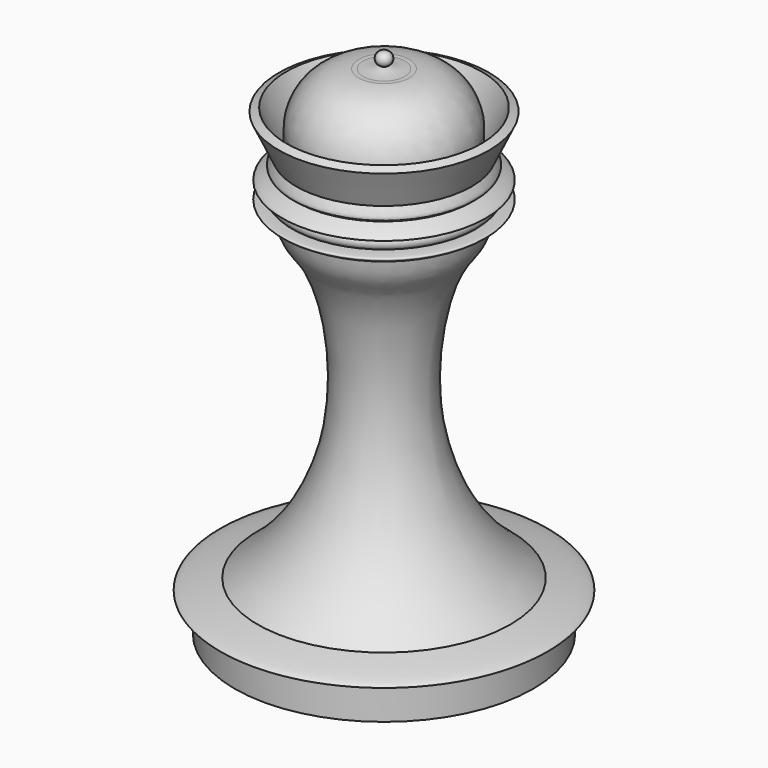
from build123d import *

# Parameters (mm, degrees)
F0_W = 22.86
F0_H = 5.08


# Not quite as in the source:
# - a fillet or chamfer that OpenCascade refuses, or shapes differently, is made with other operations: its cross-section is extruded or revolved along the edge and cut away or added
# - ends of sketch curves that miss each other by under 0.0002 mm in the source are joined


with BuildPart() as f1:
    # F0 (on Front) → F1 (revolve)
    with BuildSketch(Plane.XZ):
        with BuildLine():
            Line((0, 55.7105094194), (0, 0))
            Line((0, 0), (22.86, 0))
            add(Edge.make_bspline(
                [(22.86, 0), (21.5989604618, 0.7698820082), (20.4285707435, 1.5817251932), (19.3433039435, 2.4293450133)],
                knots=[0, 0, 0, 0, 0.0399308158, 0.0399308158, 0.0399308158, 0.0399308158], degree=3))
            add(Edge.make_bspline(
                [(19.3433039435, 2.4293450133), (2.1960366332, 15.8217786838), (8.0106373207, 47.4585030975), (12.7210086452, 48.040195095), (13.216347906, 51.9578989549)],
                knots=[0.0399308158, 0.0399308158, 0.0399308158, 0.0399308158, 0.6708396138, 0.9340401236, 0.9340401236, 0.9340401236, 0.9340401236], degree=3))
            add(Edge.make_bspline(
                [(13.216347906, 51.9578989549), (13.2835273481, 52.4892300656), (13.3343132727, 53.0894723366), (13.3667210402, 53.7746848436)],
                knots=[0.9340401236, 0.9340401236, 0.9340401236, 0.9340401236, 0.9697361905, 0.9697361905, 0.9697361905, 0.9697361905], degree=3))
            add(Edge.make_bspline(
                [(13.3667210402, 53.7746848436), (13.3941969664, 54.3556211357), (13.4084627224, 54.9976338064), (13.4083088487, 55.7105094194)],
                knots=[0.9697361905, 0.9697361905, 0.9697361905, 0.9697361905, 1, 1, 1, 1], degree=3))
            Line((13.4083088487, 55.7105094194), (0, 55.7105094194))
        make_face()
        with Locations((11.43, -2.54)):
            Rectangle(F0_W, F0_H)
        with BuildLine():
            add(Edge.make_bspline(
                [(22.86, 0), (21.5989604618, 0.7698820082), (20.4285707435, 1.5817251932), (19.3433039435, 2.4293450133)],
                knots=[0, 0, 0, 0, 0.0399308158, 0.0399308158, 0.0399308158, 0.0399308158], degree=3))
            add(Edge.make_bspline(
                [(22.86, 0), (24.0019086341, 0.246870981), (26.952558916, 0.8887774552), (22.2286200965, 1.8372453111), (19.3433039435, 2.4293450133)],
                knots=[0, 0, 0, 0, 0.3874971146, 1, 1, 1, 1], degree=3))
        make_face()
        Polygon((0, 59.5205094194), (0, 55.7105094194), (13.4083088487, 55.7105094194), (13.4083088487, 57.4333710852), (13.4083088487, 57.5264018668), (13.4083088487, 59.5205094194), (12.0004873024, 59.5205094194), align=None)
        Polygon((0, 71.0442215204), (0, 59.5205094194), (12.0004873024, 59.5205094194), (12.0004873024, 71.0442215204), (0.4261149152, 71.0442215204), align=None)
        with BuildLine():
            ThreePointArc((13.4064676104, 53.7737931527), (14.3766674197, 54.7412297913), (13.4083088487, 55.7105094194))
            add(Edge.make_bspline(
                [(13.3667210402, 53.7746848436), (13.3941969664, 54.3556211357), (13.4084627224, 54.9976338064), (13.4083088487, 55.7105094194)],
                knots=[0.9697361905, 0.9697361905, 0.9697361905, 0.9697361905, 1, 1, 1, 1], degree=3))
            add(Edge.make_bspline(
                [(13.3667210402, 53.7746848436), (13.3799703774, 53.7743877866), (13.3932198369, 53.7740906953), (13.4064676104, 53.7737931527)],
                knots=[0, 0, 0, 0, 0.0056661513, 0.0056661513, 0.0056661513, 0.0056661513], degree=3))
        make_face()
        with BuildLine():
            Line((13.4083088487, 57.4333710852), (13.4083088487, 55.7105094194))
            add(Edge.make_bspline(
                [(13.4083088487, 55.7105094194), (14.5001105526, 55.7350745123), (16.735730214, 55.7924721705), (14.5809416935, 56.8645959096), (13.4083088487, 57.4333710852)],
                knots=[0.005928529, 0.005928529, 0.005928529, 0.005928529, 0.4729046175, 0.9727722486, 0.9727722486, 0.9727722486, 0.9727722486], degree=3))
        make_face()
        with BuildLine():
            add(Edge.make_bspline(
                [(13.216347906, 51.9578989549), (13.2835273481, 52.4892300656), (13.3343132727, 53.0894723366), (13.3667210402, 53.7746848436)],
                knots=[0.9340401236, 0.9340401236, 0.9340401236, 0.9340401236, 0.9697361905, 0.9697361905, 0.9697361905, 0.9697361905], degree=3))
            add(Edge.make_bspline(
                [(13.4064676104, 53.7737931527), (14.4988968447, 53.7492573873), (16.7993068851, 53.690510951), (14.4560957231, 52.5585149788), (13.216347906, 51.9578989549)],
                knots=[0.0056661513, 0.0056661513, 0.0056661513, 0.0056661513, 0.4729046175, 1, 1, 1, 1], degree=3))
            ThreePointArc((13.4064676104, 53.7737931527), (13.3865897487, 53.7740349992), (13.3667210402, 53.7746848436))
        make_face()
        with BuildLine():
            Line((0, 73.3851119876), (0, 71.0442215204))
            Line((0, 71.0442215204), (0.4261149152, 71.0442215204))
            Line((0.4261149152, 71.0442215204), (0.4261149152, 71.5328380466))
            ThreePointArc((0.4261149152, 71.5328380466), (1.1047984107, 72.6641196839), (0, 73.3851119876))
        make_face()
        Polygon((14.9355589143, 65.8147908034), (12.0004873024, 59.5205094194), (13.4083088487, 59.5205094194), (16.0919348108, 65.2755638671), align=None)
        with BuildLine():
            add(Edge.make_bspline(
                [(13.3667210402, 53.7746848436), (13.3799703774, 53.7743877866), (13.3932198369, 53.7740906953), (13.4064676104, 53.7737931527)],
                knots=[0, 0, 0, 0, 0.0056661513, 0.0056661513, 0.0056661513, 0.0056661513], degree=3))
            ThreePointArc((13.3667210402, 53.7746848436), (13.3865897487, 53.7740349992), (13.4064676104, 53.7737931527))
        make_face()
        with BuildLine():
            add(Edge.make_bspline(
                [(13.4083088487, 59.5205094194), (13.7410667142, 58.9220634461), (14.2957709416, 57.9244596453), (13.6619222311, 57.6401563363), (13.4083088487, 57.5264018668)],
                knots=[0, 0, 0, 0, 0.5998834136, 1, 1, 1, 1], degree=3))
            Line((13.4083088487, 59.5205094194), (13.4083088487, 57.5264018668))
        make_face()
    revolve(axis=Axis((0, 0, 65.2355094194), (0, 0, -1)))

    # F2: fillet of radius 8.128 on 2 edges, made by hand

    # F2_s1 → F2_t2 (revolve)
    with BuildSketch(Plane.XZ):
        with BuildLine():
            ThreePointArc((3.2017597302, 71.0442215204), (1.7925977231, 71.1673076272), (0.4261149152, 71.5328380466))
            Line((0.4261149152, 71.5328380466), (0.4261149152, 71.0442215204))
            Line((0.4261149152, 71.0442215204), (3.2017597302, 71.0442215204))
        make_face()
    revolve(axis=Axis((0, 0, 71.0442215204), (0, 0, -1)))

    # F2_s3 → F2_t4 (revolve, cut)
    with BuildSketch(Plane.XZ):
        with BuildLine():
            ThreePointArc((12.0004873024, 62.9162215204), (9.6198512199, 68.6635854379), (3.8724873024, 71.0442215204))
            Line((3.8724873024, 71.0442215204), (12.0004873024, 71.0442215204))
            Line((12.0004873024, 71.0442215204), (12.0004873024, 62.9162215204))
        make_face()
    revolve(axis=Axis((0, 0, 71.0442215204), (0, 0, -1)), mode=Mode.SUBTRACT)


solid = f1.part
